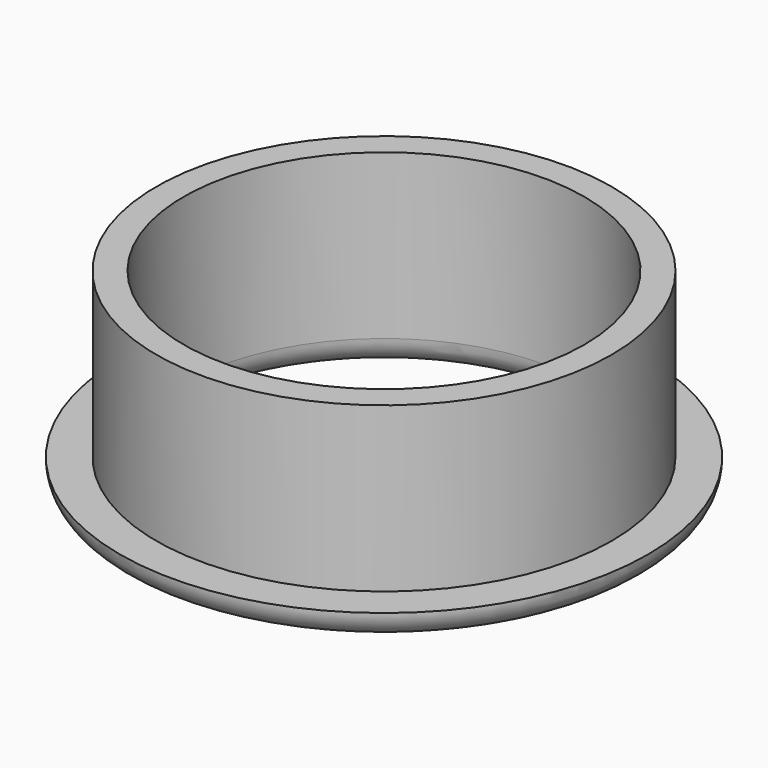
from build123d import *

# Parameters (mm, degrees)
F0_R     = 25
F1_DEPTH = 18
F2_R     = 29
F3_DEPTH = 3
F4_R     = 22
F5_DEPTH = 21.001
F6_R     = 2.99999


# Not quite as in the source:
# - a fillet or chamfer is up to 0.001 mm smaller than in the source, because OpenCascade refuses the exact size


with BuildPart() as f1:
    # F0 (on Top) → F1 (new body)
    with BuildSketch(Plane.XY):
        Circle(F0_R)
    extrude(amount=F1_DEPTH)

    # F2 (on Top) → F3 (join)
    with BuildSketch(Plane.XY):
        Circle(F2_R)
    extrude(amount=-F3_DEPTH)

    # F4 (on face) → F5 (cut, through all)
    with BuildSketch(Plane.XY.offset(18)):
        Circle(F4_R)
    extrude(amount=-F5_DEPTH, mode=Mode.SUBTRACT)

    # F6 (radius 3 in the source; OpenCascade refuses exactly that, so slightly less here)
    f6_edges = [f1.edges().sort_by_distance(p)[0] for p in [
        (-22, 0, -3),
        (-29, 0, -3),
    ]]
    fillet(f6_edges, radius=F6_R)


solid = f1.part
